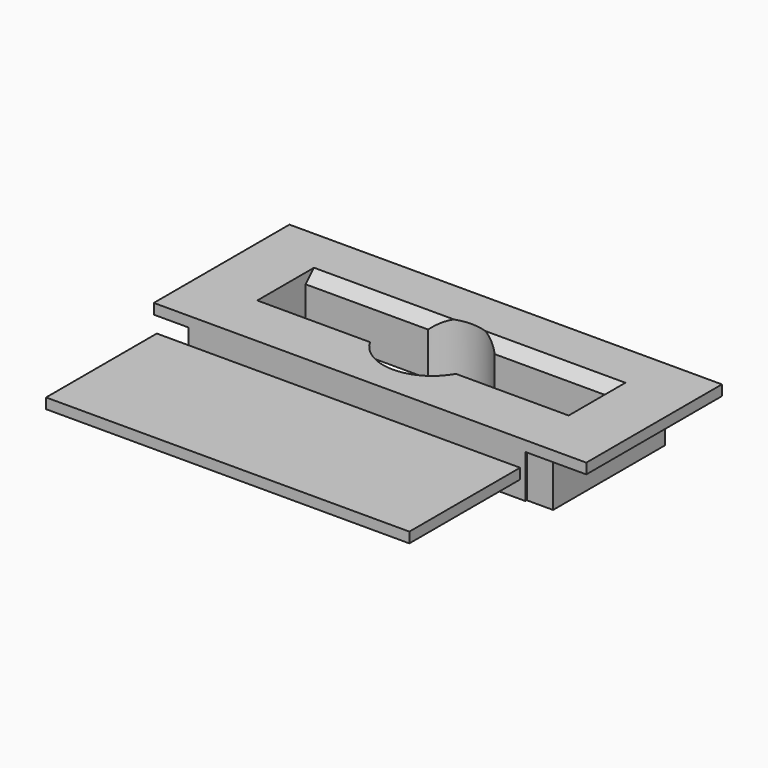
from build123d import *

# Parameters (mm, degrees)
F0_W         = 18
F0_H         = 1.6
F1_DEPTH     = 0.6
F0_W_2       = 21
F0_H_2       = 8
F2_DEPTH     = 4
F3_T4_DEPTH  = 18.3473034272
F3_T9_DEPTH  = 18.3473034272
F3_T14_ANGLE = 359.64
F4_SIZE      = 0.59999
F5_DEPTH     = 2.5


# Not quite as in the source:
# - a fillet or chamfer that OpenCascade refuses, or shapes differently, is made with other operations: its cross-section is extruded or revolved along the edge and cut away or added
# - a fillet or chamfer is up to 0.001 mm smaller than in the source, because OpenCascade refuses the exact size
# - a feature of the source that left no trace in its solid (it failed there, or was rolled back) is left out


with BuildPart() as f1:
    # F0 (on Top) → F1 (new body)
    with BuildSketch(Plane.XY):
        Polygon((-17.0167625099, -0.2778713822), (-20.5167625099, -0.2778713822), (-20.5167625099, -10.0778713822), (-18.5167625099, -10.0778713822), (-18.5167625099, -1.8778713822), (-17.0167625099, -1.8778713822), align=None)
        with Locations((-8.0167625099, -1.0778713822)):
            Rectangle(F0_W, F0_H)
        Polygon((4.4832374901, -0.2778713822), (0.9832374901, -0.2778713822), (0.9832374901, -1.8778713822), (2.4832374901, -1.8778713822), (2.4832374901, -9.9778713822), (0.9832374901, -9.9778713822), (0.9832374901, -10.0778713822), (4.4832374901, -10.0778713822), align=None)
        Polygon((-17.0167625099, -3.4778713822), (-17.0167625099, -1.8778713822), (-18.5167625099, -1.8778713822), (-18.5167625099, -10.0778713822), (-17.0167625099, -10.0778713822), (-17.0167625099, -6.9778713822), align=None)
        with BuildLine():
            Line((-17.0167625099, -6.9778713822), (-17.0167625099, -10.0778713822))
            Line((-17.0167625099, -10.0778713822), (0.9832374901, -10.0778713822))
            Line((0.9832374901, -10.0778713822), (0.9832374901, -9.9778713822))
            Line((0.9832374901, -9.9778713822), (0.9832374901, -6.9778713822))
            Line((0.9832374901, -6.9778713822), (-5.5343241925, -6.9778713822))
            ThreePointArc((-5.5343241925, -6.9778713822), (-8.0167625099, -8.4278713822), (-10.4992008274, -6.9778713822))
            Line((-10.4992008274, -6.9778713822), (-17.0167625099, -6.9778713822))
        make_face()
        Polygon((2.4832374901, -1.8778713822), (0.9832374901, -1.8778713822), (0.9832374901, -3.4778713822), (0.9832374901, -6.9778713822), (0.9832374901, -9.9778713822), (2.4832374901, -9.9778713822), align=None)
        with BuildLine():
            Line((0.9832374901, -1.8778713822), (-17.0167625099, -1.8778713822))
            Line((-17.0167625099, -1.8778713822), (-17.0167625099, -3.4778713822))
            Line((-17.0167625099, -3.4778713822), (-9.9435473967, -3.4778713822))
            ThreePointArc((-9.9435473967, -3.4778713822), (-8.0167625099, -2.7278713822), (-6.0899776231, -3.4778713822))
            Line((-6.0899776231, -3.4778713822), (0.9832374901, -3.4778713822))
            Line((0.9832374901, -3.4778713822), (0.9832374901, -1.8778713822))
        make_face()
    extrude(amount=F1_DEPTH)

    # F0 (on Top) → F2 (join)
    with BuildSketch(Plane.XY):
        with BuildLine():
            Line((-17.0167625099, -6.9778713822), (-17.0167625099, -10.0778713822))
            Line((-17.0167625099, -10.0778713822), (0.9832374901, -10.0778713822))
            Line((0.9832374901, -10.0778713822), (0.9832374901, -9.9778713822))
            Line((0.9832374901, -9.9778713822), (0.9832374901, -6.9778713822))
            Line((0.9832374901, -6.9778713822), (-5.5343241925, -6.9778713822))
            ThreePointArc((-5.5343241925, -6.9778713822), (-8.0167625099, -8.4278713822), (-10.4992008274, -6.9778713822))
            Line((-10.4992008274, -6.9778713822), (-17.0167625099, -6.9778713822))
        make_face()
    extrude(amount=-F2_DEPTH)

    # F3: chamfer of 4.6 on 3 edges, made by hand


with BuildPart() as f1b:
    # F0 (on Top) → F1, piece 2 (new body)
    with BuildSketch(Plane.XY):
        with Locations((-8.0406878591, -16.3323699534)):
            Rectangle(F0_W_2, F0_H_2)
    extrude(amount=F1_DEPTH)


with BuildPart() as f3_tool2:
    # F3_s3 → F3_t4 (new body)
    with BuildSketch(Plane.YZ.offset(1.3305409172)):
        Polygon((-11.5778713822, -4), (-6.9778713822, 0.6), (-6.9778713822, -4), align=None)
    extrude(amount=-F3_T4_DEPTH)

    split(bisect_by=Plane.YZ.offset(0.9832374901), keep=Keep.BOTTOM)


with BuildPart() as f1_1:
    add(f1.part)

    # F3_t1: cut F3_tool2
    add(f3_tool2.part, mode=Mode.SUBTRACT)


with BuildPart() as f3_tool7:
    # F3_s8 → F3_t9 (new body)
    with BuildSketch(Plane.YZ.offset(0.9832374901)):
        Polygon((-11.5778713822, -4), (-6.9778713822, 0.6), (-6.9778713822, -4), align=None)
    extrude(amount=-F3_T9_DEPTH)

    split(bisect_by=Plane.YZ.offset(-17.0167625099), keep=Keep.TOP)


with BuildPart() as f1_2:
    add(f1_1.part)

    # F3_t6: cut F3_tool7
    add(f3_tool7.part, mode=Mode.SUBTRACT)


with BuildPart() as f3_tool12:
    # F3_s13 → F3_t14 (revolve)
    with BuildSketch(Plane(origin=(-7.9991601035, 0.0251301853, 0), x_dir=(0, 0, 1), z_dir=(-0.9999950652, 0.0031415875, 0))):
        Polygon((0.6, -2.7530292173), (-4, 1.8469707827), (-4, -2.7530292173), align=None)
    revolve(axis=Axis((-8.0167625099, -5.5778713822, -4), (0, 0, -1)), revolution_arc=F3_T14_ANGLE)

    split(bisect_by=Plane.XZ.offset(3.4778713822), keep=Keep.TOP)


with BuildPart() as f1_3:
    add(f1_2.part)

    # F3_t11: cut F3_tool12
    add(f3_tool12.part, mode=Mode.SUBTRACT)

    # F4 (size 0.6 in the source; OpenCascade refuses exactly that, so slightly less here)
    f4_edges = [f1_3.edges().sort_by_distance(p)[0] for p in [
        (-13.480155, -3.477871, 0.6),
        (-2.55337, -3.477871, 0.6),
    ]]
    chamfer(f4_edges, length=F4_SIZE)

    # F0 (on Top) → F5 (join)
    with BuildSketch(Plane.XY):
        Polygon((-17.0167625099, -3.4778713822), (-17.0167625099, -1.8778713822), (-18.5167625099, -1.8778713822), (-18.5167625099, -10.0778713822), (-17.0167625099, -10.0778713822), (-17.0167625099, -6.9778713822), align=None)
        with BuildLine():
            Line((0.9832374901, -1.8778713822), (-17.0167625099, -1.8778713822))
            Line((-17.0167625099, -1.8778713822), (-17.0167625099, -3.4778713822))
            Line((-17.0167625099, -3.4778713822), (-9.9435473967, -3.4778713822))
            ThreePointArc((-9.9435473967, -3.4778713822), (-8.0167625099, -2.7278713822), (-6.0899776231, -3.4778713822))
            Line((-6.0899776231, -3.4778713822), (0.9832374901, -3.4778713822))
            Line((0.9832374901, -3.4778713822), (0.9832374901, -1.8778713822))
        make_face()
        Polygon((2.4832374901, -1.8778713822), (0.9832374901, -1.8778713822), (0.9832374901, -3.4778713822), (0.9832374901, -6.9778713822), (0.9832374901, -9.9778713822), (2.4832374901, -9.9778713822), align=None)
    extrude(amount=-F5_DEPTH)


solid = Compound([f1b.part, f1_3.part])
